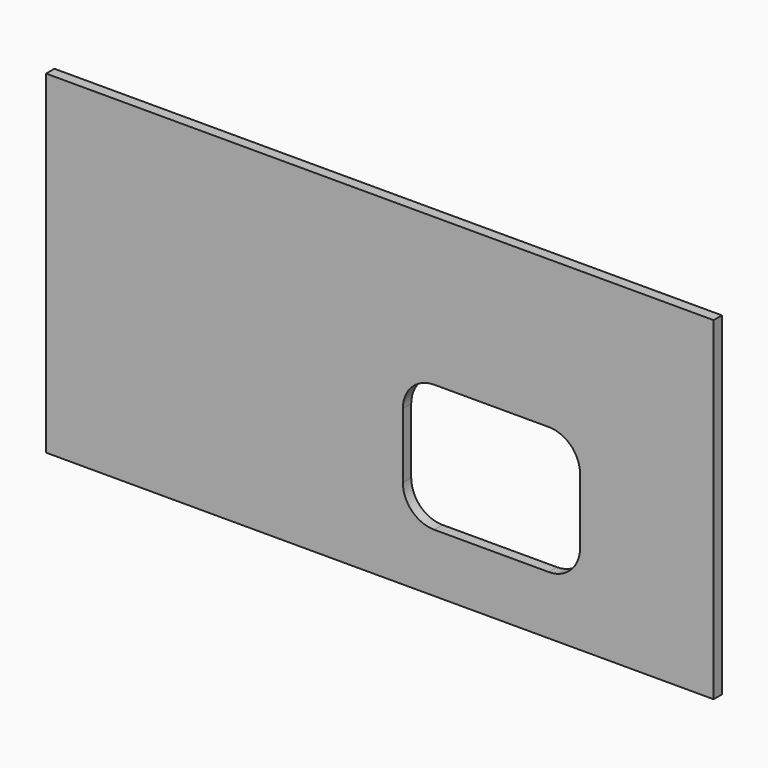
from build123d import *

# Parameters (mm, degrees)
F0_W     = 101.6
F0_H     = 50.8
F1_DEPTH = 1.5875


# Not quite as in the source:
# - a length typed as a fraction of an inch, garbled in the dataset ("3 / 203.2 mm" for 3/8 in), is restored


with BuildPart() as f1:
    # F0 (on Front) → F1 (new body)
    with BuildSketch(Plane.XZ):
        with Locations((50.8, 25.4)):
            Rectangle(F0_W, F0_H)
        with BuildLine():
            ThreePointArc((81.28, 13.6525), (79.8850960454, 10.2849039546), (76.5175, 8.89))
            Line((76.5175, 8.89), (59.0677, 8.89))
            ThreePointArc((59.0677, 8.89), (55.7001039546, 10.2849039546), (54.3052, 13.6525))
            Line((54.3052, 13.6525), (54.3052, 23.5585))
            ThreePointArc((54.3052, 23.5585), (55.7001039546, 26.9260960454), (59.0677, 28.321))
            Line((59.0677, 28.321), (76.5175, 28.321))
            ThreePointArc((76.5175, 28.321), (79.8850960454, 26.9260960454), (81.28, 23.5585))
            Line((81.28, 23.5585), (81.28, 13.6525))
        make_face(mode=Mode.SUBTRACT)
    extrude(amount=F1_DEPTH)


solid = f1.part
